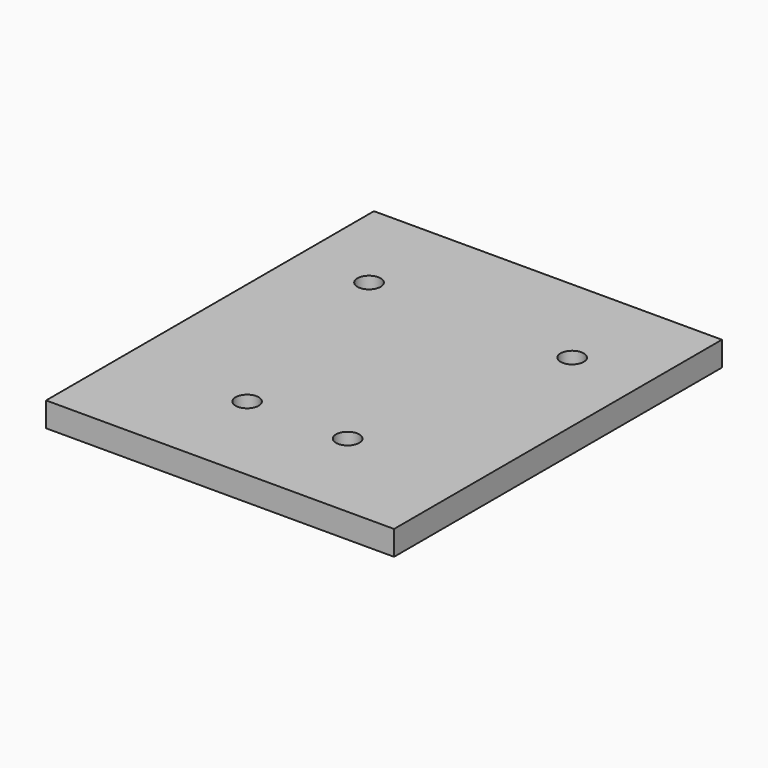
from build123d import *

# Parameters (mm, degrees)
F0_W     = 90
F0_H     = 106
F1_DEPTH = 6.35
F2_R     = 3
F3_DEPTH = 25


# Not quite as in the source:
# - a length typed as a fraction of an inch, garbled in the dataset ("3 / 203.2 mm" for 3/8 in), is restored


with BuildPart() as f1:
    # F0 (on Top) → F1 (new body)
    with BuildSketch(Plane.XY):
        with Locations((3.2195534329, 9.4163397849)):
            Rectangle(F0_W, F0_H)
    extrude(amount=F1_DEPTH)

    # F2 (on face) → F3 (cut)
    with BuildSketch(Plane.XY.offset(6.35)):
        with Locations((-23.0504465671, 37.4163397849)):
            Circle(F2_R)
        with Locations((29.4895534329, 37.4163397849)):
            Circle(F2_R)
        with Locations((-9.7804465671, -18.5836602151)):
            Circle(F2_R)
        with Locations((16.2195534329, -18.5836602151)):
            Circle(F2_R)
    extrude(amount=-F3_DEPTH, mode=Mode.SUBTRACT)


solid = f1.part
